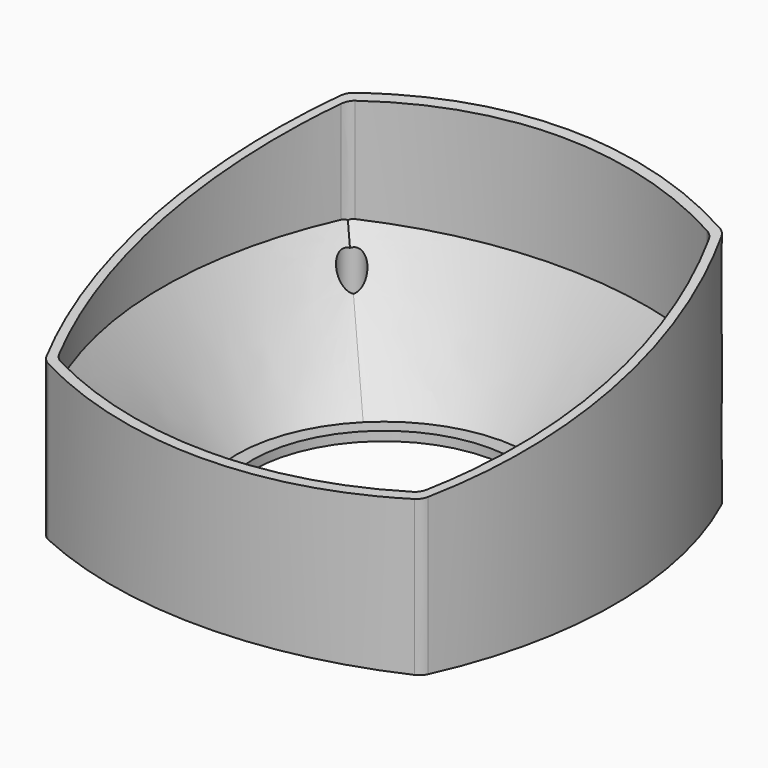
from build123d import *

# Parameters (mm, degrees)
F1_DEPTH        = 80
F2_R            = 1379.3418086479
F3_DEPTH        = 390
F0_R            = 47.8625
F7_DEPTH        = 40
F8_R            = 47.8625
F10_R           = 42.8625
F11_DEPTH       = 3
F14_DEPTH       = 31
F16_DEPTH       = 25
F17_R           = 5
F20_D           = 4
F20_START       = 24.8328661
F20_CBORE_D     = 8
F20_CBORE_DEPTH = 5
F21_R           = 2
F22_DEPTH       = 3
F23_R           = 12.5
F24_DEPTH       = 249
F25_R           = 125
F26_DEPTH       = 125


# Not quite as in the source:
# - a feature names something its author has since deleted; it is built from what else it names


with BuildPart() as f1:
    # F0 (on Top) → F1 (new body, symmetric)
    with BuildSketch(Plane.XY):
        with BuildLine():
            ThreePointArc((61.2553872941, -61.2553872941), (75.039376183, 0), (61.2553872941, 61.2553872941))
            ThreePointArc((61.2553872941, 61.2553872941), (0, 75.039376183), (-61.2553872941, 61.2553872941))
            ThreePointArc((-61.2553872941, 61.2553872941), (-75.039376183, 0), (-61.2553872941, -61.2553872941))
            ThreePointArc((-61.2553872941, -61.2553872941), (0, -75.039376183), (61.2553872941, -61.2553872941))
        make_face()
        with BuildLine():
            ThreePointArc((-59, 59), (0, 72.039376183), (59, 59))
            ThreePointArc((59, 59), (72.039376183, 0), (59, -59))
            ThreePointArc((59, -59), (0, -72.039376183), (-59, -59))
            ThreePointArc((-59, -59), (-72.039376183, 0), (-59, 59))
        make_face(mode=Mode.SUBTRACT)
    extrude(amount=F1_DEPTH, both=True)

    # F2 (on Right) → F3 (cut, symmetric)
    with BuildSketch(Plane.YZ):
        with Locations((-294.0411567688, 1407.0612192154)):
            Circle(F2_R)
        with Locations((-294.0411567688, -1407.0612192154)):
            Circle(F2_R)
    extrude(amount=F3_DEPTH, both=True, mode=Mode.SUBTRACT)

    # F6 (on Top) + F0 (on Top) → F7 (join, symmetric)
    with BuildSketch(Plane.XY):
        with BuildLine():
            ThreePointArc((61.2553872941, -61.2553872941), (75.039376183, 0), (61.2553872941, 61.2553872941))
            ThreePointArc((61.2553872941, 61.2553872941), (0, 75.039376183), (-61.2553872941, 61.2553872941))
            ThreePointArc((-61.2553872941, 61.2553872941), (-75.039376183, 0), (-61.2553872941, -61.2553872941))
            ThreePointArc((-61.2553872941, -61.2553872941), (0, -75.039376183), (61.2553872941, -61.2553872941))
        make_face()
        with BuildLine():
            ThreePointArc((-59, 59), (0, 72.039376183), (59, 59))
            ThreePointArc((59, 59), (72.039376183, 0), (59, -59))
            ThreePointArc((59, -59), (0, -72.039376183), (-59, -59))
            ThreePointArc((-59, -59), (-72.039376183, 0), (-59, 59))
        make_face(mode=Mode.SUBTRACT)
        with BuildLine():
            ThreePointArc((59, -59), (72.039376183, 0), (59, 59))
            ThreePointArc((59, 59), (0, 72.039376183), (-59, 59))
            ThreePointArc((-59, 59), (-72.039376183, 0), (-59, -59))
            ThreePointArc((-59, -59), (0, -72.039376183), (59, -59))
        make_face()
    with BuildSketch(Plane.XY):
        with BuildLine():
            ThreePointArc((59, -59), (72.039376183, 0), (59, 59))
            ThreePointArc((59, 59), (0, 72.039376183), (-59, 59))
            ThreePointArc((-59, 59), (-72.039376183, 0), (-59, -59))
            ThreePointArc((-59, -59), (0, -72.039376183), (59, -59))
        make_face()
        Circle(F0_R, mode=Mode.SUBTRACT)
    extrude(amount=F7_DEPTH, both=True)

    # F5 (on offset) → F9 section 0
    with BuildSketch(Plane.XY.offset(40)):
        with BuildLine():
            ThreePointArc((59, -59), (72.039376183, 0), (59, 59))
            ThreePointArc((59, 59), (0, 72.039376183), (-59, 59))
            ThreePointArc((-59, 59), (-72.039376183, 0), (-59, -59))
            ThreePointArc((-59, -59), (0, -72.039376183), (59, -59))
        make_face()
    # F8 (on Top) → F9 section 1
    with BuildSketch(Plane.XY):
        Circle(F8_R)
    loft(mode=Mode.SUBTRACT)

    # F10 (on face) → F11 (cut)
    with BuildSketch(Plane.XY):
        Circle(F10_R)
    extrude(amount=-F11_DEPTH, mode=Mode.SUBTRACT)

    # F13 (on offset) → F14 (cut)
    with BuildSketch(Plane.XY.offset(-3)):
        with BuildLine():
            ThreePointArc((59, -59), (72.039376183, 0), (59, 59))
            ThreePointArc((59, 59), (0, 72.039376183), (-59, 59))
            ThreePointArc((-59, 59), (-72.039376183, 0), (-59, -59))
            ThreePointArc((-59, -59), (0, -72.039376183), (59, -59))
        make_face()
    extrude(amount=-F14_DEPTH, mode=Mode.SUBTRACT)

    # F15 (on face) → F16 (cut)
    with BuildSketch(Plane(origin=(0, 0, -40), x_dir=(1, 0, 0), z_dir=(0, 0, -1))):
        with BuildLine():
            Line((-1, 60.9918027279), (-1, 62.4919994879))
            ThreePointArc((-1, 62.4919994879), (-44.1941738242, 44.1941738242), (-62.4919994879, 1))
            Line((-62.4919994879, 1), (-60.9918027279, 1))
            ThreePointArc((-60.9918027279, 1), (-43.1335136524, 43.1335136524), (-1, 60.9918027279))
        make_face()
        with BuildLine():
            Line((-1, 55.9910707167), (-1, 57.4913036902))
            ThreePointArc((-1, 57.4913036902), (-40.6586399182, 40.6586399182), (-57.4913036902, 1))
            Line((-57.4913036902, 1), (-55.9910707167, 1))
            ThreePointArc((-55.9910707167, 1), (-39.5979797464, 39.5979797464), (-1, 55.9910707167))
        make_face()
        with BuildLine():
            Line((-1, 50.9901951359), (-1, 52.4904753265))
            ThreePointArc((-1, 52.4904753265), (-37.1231060123, 37.1231060123), (-52.4904753265, 1))
            Line((-52.4904753265, 1), (-50.9901951359, 1))
            ThreePointArc((-50.9901951359, 1), (-36.0624458405, 36.0624458405), (-1, 50.9901951359))
        make_face()
        with BuildLine():
            Line((-1, 45.9891291503), (-1, 47.4894725176))
            ThreePointArc((-1, 47.4894725176), (-33.5875721064, 33.5875721064), (-47.4894725176, 1))
            Line((-47.4894725176, 1), (-45.9891291503, 1))
            ThreePointArc((-45.9891291503, 1), (-32.5269119346, 32.5269119346), (-1, 45.9891291503))
        make_face()
        with BuildLine():
            Line((-1, 40.9878030638), (-1, 42.4882336653))
            ThreePointArc((-1, 42.4882336653), (-30.0520382004, 30.0520382004), (-42.4882336653, 1))
            Line((-42.4882336653, 1), (-40.9878030638, 1))
            ThreePointArc((-40.9878030638, 1), (-28.9913780286, 28.9913780286), (-1, 40.9878030638))
        make_face()
        with BuildLine():
            Line((-1, 35.9861084309), (-1, 37.4866642955))
            ThreePointArc((-1, 37.4866642955), (-26.5165042945, 26.5165042945), (-37.4866642955, 1))
            Line((-37.4866642955, 1), (-35.9861084309, 1))
            ThreePointArc((-35.9861084309, 1), (-25.4558441227, 25.4558441227), (-1, 35.9861084309))
        make_face()
        with BuildLine():
            Line((35.9861084309, 1), (37.4866642955, 1))
            ThreePointArc((37.4866642955, 1), (26.5165042945, 26.5165042945), (1, 37.4866642955))
            Line((1, 37.4866642955), (1, 35.9861084309))
            ThreePointArc((1, 35.9861084309), (25.4558441227, 25.4558441227), (35.9861084309, 1))
        make_face()
        with BuildLine():
            Line((40.9878030638, 1), (42.4882336653, 1))
            ThreePointArc((42.4882336653, 1), (30.0520382004, 30.0520382004), (1, 42.4882336653))
            Line((1, 42.4882336653), (1, 40.9878030638))
            ThreePointArc((1, 40.9878030638), (28.9913780286, 28.9913780286), (40.9878030638, 1))
        make_face()
        with BuildLine():
            Line((45.9891291503, 1), (47.4894725176, 1))
            ThreePointArc((47.4894725176, 1), (33.5875721064, 33.5875721064), (1, 47.4894725176))
            Line((1, 47.4894725176), (1, 45.9891291503))
            ThreePointArc((1, 45.9891291503), (32.5269119346, 32.5269119346), (45.9891291503, 1))
        make_face()
        with BuildLine():
            Line((50.9901951359, 1), (52.4904753265, 1))
            ThreePointArc((52.4904753265, 1), (37.1231060123, 37.1231060123), (1, 52.4904753265))
            Line((1, 52.4904753265), (1, 50.9901951359))
            ThreePointArc((1, 50.9901951359), (36.0624458405, 36.0624458405), (50.9901951359, 1))
        make_face()
        with BuildLine():
            Line((55.9910707167, 1), (57.4913036902, 1))
            ThreePointArc((57.4913036902, 1), (40.6586399182, 40.6586399182), (1, 57.4913036902))
            Line((1, 57.4913036902), (1, 55.9910707167))
            ThreePointArc((1, 55.9910707167), (39.5979797464, 39.5979797464), (55.9910707167, 1))
        make_face()
        with BuildLine():
            Line((60.9918027279, 1), (62.4919994879, 1))
            ThreePointArc((62.4919994879, 1), (44.1941738242, 44.1941738242), (1, 62.4919994879))
            Line((1, 62.4919994879), (1, 60.9918027279))
            ThreePointArc((1, 60.9918027279), (43.1335136524, 43.1335136524), (60.9918027279, 1))
        make_face()
        with BuildLine():
            ThreePointArc((1, -37.4866642955), (26.5165042945, -26.5165042945), (37.4866642955, -1))
            Line((37.4866642955, -1), (35.9861084309, -1))
            ThreePointArc((35.9861084309, -1), (25.4558441227, -25.4558441227), (1, -35.9861084309))
            Line((1, -35.9861084309), (1, -37.4866642955))
        make_face()
        with BuildLine():
            ThreePointArc((-37.4866642955, -1), (-26.5165042945, -26.5165042945), (-1, -37.4866642955))
            Line((-1, -37.4866642955), (-1, -35.9861084309))
            ThreePointArc((-1, -35.9861084309), (-25.4558441227, -25.4558441227), (-35.9861084309, -1))
            Line((-35.9861084309, -1), (-37.4866642955, -1))
        make_face()
        with BuildLine():
            ThreePointArc((-42.4882336653, -1), (-30.0520382004, -30.0520382004), (-1, -42.4882336653))
            Line((-1, -42.4882336653), (-1, -40.9878030638))
            ThreePointArc((-1, -40.9878030638), (-28.9913780286, -28.9913780286), (-40.9878030638, -1))
            Line((-40.9878030638, -1), (-42.4882336653, -1))
        make_face()
        with BuildLine():
            ThreePointArc((1, -42.4882336653), (30.0520382004, -30.0520382004), (42.4882336653, -1))
            Line((42.4882336653, -1), (40.9878030638, -1))
            ThreePointArc((40.9878030638, -1), (28.9913780286, -28.9913780286), (1, -40.9878030638))
            Line((1, -40.9878030638), (1, -42.4882336653))
        make_face()
        with BuildLine():
            ThreePointArc((1, -47.4894725176), (33.5875721064, -33.5875721064), (47.4894725176, -1))
            Line((47.4894725176, -1), (45.9891291503, -1))
            ThreePointArc((45.9891291503, -1), (32.5269119346, -32.5269119346), (1, -45.9891291503))
            Line((1, -45.9891291503), (1, -47.4894725176))
        make_face()
        with BuildLine():
            ThreePointArc((-47.4894725176, -1), (-33.5875721064, -33.5875721064), (-1, -47.4894725176))
            Line((-1, -47.4894725176), (-1, -45.9891291503))
            ThreePointArc((-1, -45.9891291503), (-32.5269119346, -32.5269119346), (-45.9891291503, -1))
            Line((-45.9891291503, -1), (-47.4894725176, -1))
        make_face()
        with BuildLine():
            ThreePointArc((-52.4904753265, -1), (-37.1231060123, -37.1231060123), (-1, -52.4904753265))
            Line((-1, -52.4904753265), (-1, -50.9901951359))
            ThreePointArc((-1, -50.9901951359), (-36.0624458405, -36.0624458405), (-50.9901951359, -1))
            Line((-50.9901951359, -1), (-52.4904753265, -1))
        make_face()
        with BuildLine():
            ThreePointArc((1, -52.4904753265), (37.1231060123, -37.1231060123), (52.4904753265, -1))
            Line((52.4904753265, -1), (50.9901951359, -1))
            ThreePointArc((50.9901951359, -1), (36.0624458405, -36.0624458405), (1, -50.9901951359))
            Line((1, -50.9901951359), (1, -52.4904753265))
        make_face()
        with BuildLine():
            ThreePointArc((1, -57.4913036902), (40.6586399182, -40.6586399182), (57.4913036902, -1))
            Line((57.4913036902, -1), (55.9910707167, -1))
            ThreePointArc((55.9910707167, -1), (39.5979797464, -39.5979797464), (1, -55.9910707167))
            Line((1, -55.9910707167), (1, -57.4913036902))
        make_face()
        with BuildLine():
            ThreePointArc((-57.4913036902, -1), (-40.6586399182, -40.6586399182), (-1, -57.4913036902))
            Line((-1, -57.4913036902), (-1, -55.9910707167))
            ThreePointArc((-1, -55.9910707167), (-39.5979797464, -39.5979797464), (-55.9910707167, -1))
            Line((-55.9910707167, -1), (-57.4913036902, -1))
        make_face()
        with BuildLine():
            ThreePointArc((-62.4919994879, -1), (-44.1941738242, -44.1941738242), (-1, -62.4919994879))
            Line((-1, -62.4919994879), (-1, -60.9918027279))
            ThreePointArc((-1, -60.9918027279), (-43.1335136524, -43.1335136524), (-60.9918027279, -1))
            Line((-60.9918027279, -1), (-62.4919994879, -1))
        make_face()
        with BuildLine():
            ThreePointArc((1, -62.4919994879), (44.1941738242, -44.1941738242), (62.4919994879, -1))
            Line((62.4919994879, -1), (60.9918027279, -1))
            ThreePointArc((60.9918027279, -1), (43.1335136524, -43.1335136524), (1, -60.9918027279))
            Line((1, -60.9918027279), (1, -62.4919994879))
        make_face()
    extrude(amount=-F16_DEPTH, mode=Mode.SUBTRACT)

    # F17
    f17_edges = [f1.edges().sort_by_distance(p)[0] for p in [
        (-61.255387, 61.255387, 0),
        (-61.255387, -61.255387, 0),
        (61.255387, 61.255387, 0),
        (61.255387, -61.255387, 0),
        (-59, 59, 56.832446),
        (59, 59, 56.832446),
        (-59, -59, 43.946273),
        (59, -59, 43.946273),
        (59, -59, -43.946273),
        (-59, -59, -43.946273),
        (-59, 59, -56.832446),
        (59, 59, -56.832446),
    ]]
    fillet(f17_edges, radius=F17_R)

    # F20 (through all)
    # its depths count from where the whole tool has entered the part; down to there all is cleared
    with Locations(Plane.XY.offset(50).offset(-F20_START)):
        with Locations((-52.5, 52.5), (52.5, 52.5), (52.5, -52.5), (-52.5, -52.5)):
            CounterBoreHole(F20_D / 2, F20_CBORE_D / 2, F20_CBORE_DEPTH)

    # F21 (on face) → F22 (cut)
    with BuildSketch(Plane(origin=(0, 0, -40), x_dir=(1, 0, 0), z_dir=(0, 0, -1))):
        Polygon((-50.7679491924, 55.5), (-54.2320508076, 55.5), (-55.9641016151, 52.5), (-54.2320508076, 49.5), (-50.7679491924, 49.5), (-49.0358983849, 52.5), align=None)
        with Locations((-52.5, 52.5)):
            Circle(F21_R, mode=Mode.SUBTRACT)
        Polygon((54.2320508076, 55.5), (50.7679491924, 55.5), (49.0358983849, 52.5), (50.7679491924, 49.5), (54.2320508076, 49.5), (55.9641016151, 52.5), align=None)
        with Locations((52.5, 52.5)):
            Circle(F21_R, mode=Mode.SUBTRACT)
        Polygon((54.2320508076, -49.5), (50.7679491924, -49.5), (49.0358983849, -52.5), (50.7679491924, -55.5), (54.2320508076, -55.5), (55.9641016151, -52.5), align=None)
        with Locations((52.5, -52.5)):
            Circle(F21_R, mode=Mode.SUBTRACT)
        Polygon((-50.7679491924, -49.5), (-54.2320508076, -49.5), (-55.9641016151, -52.5), (-54.2320508076, -55.5), (-50.7679491924, -55.5), (-49.0358983849, -52.5), align=None)
        with Locations((-52.5, -52.5)):
            Circle(F21_R, mode=Mode.SUBTRACT)
    extrude(amount=-F22_DEPTH, mode=Mode.SUBTRACT)

    # F23 (on Right) → F24 (cut)
    with BuildSketch(Plane.YZ):
        with Locations((-40, -20)):
            Circle(F23_R)
    extrude(amount=F24_DEPTH, mode=Mode.SUBTRACT)

    # F25 (on offset) → F26 (cut)
    with BuildSketch(Plane.XY.offset(-3)):
        Circle(F25_R)
    extrude(amount=-F26_DEPTH, mode=Mode.SUBTRACT)


solid = f1.part
